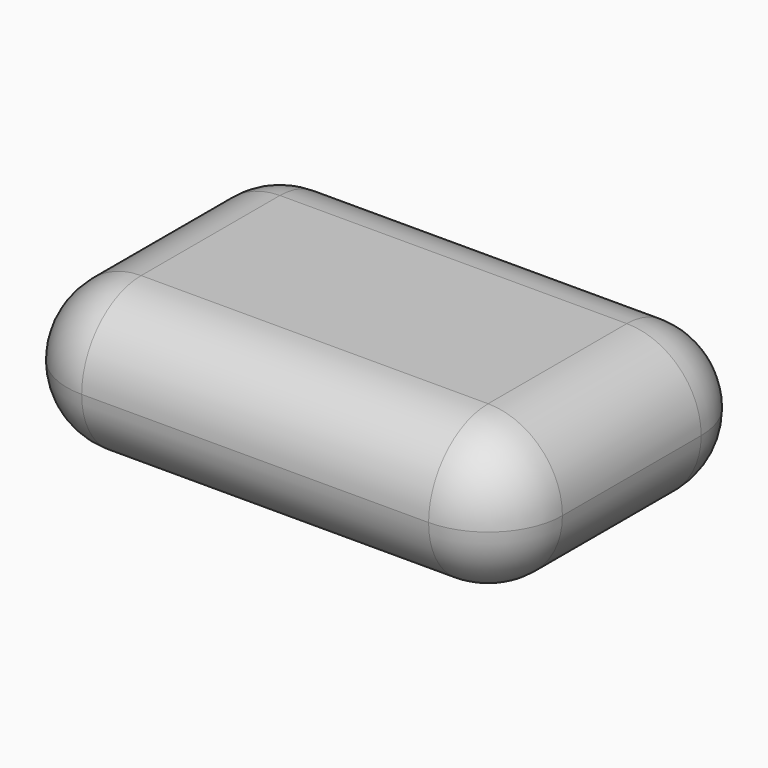
from build123d import *

# Parameters (mm, degrees)
F0_W     = 508
F0_H     = 330.2
F1_DEPTH = 152.4
F2_R     = 76.19999


# Not quite as in the source:
# - a fillet or chamfer is up to 0.001 mm smaller than in the source, because OpenCascade refuses the exact size


with BuildPart() as f1:
    # F0 (on Top) → F1 (new body)
    with BuildSketch(Plane.XY):
        Rectangle(F0_W, F0_H)
    extrude(amount=F1_DEPTH)

    # F2 (radius 76.2 in the source; OpenCascade refuses exactly that, so slightly less here)
    f2_edges = [f1.edges().sort_by_distance(p)[0] for p in [
        (254, 0, 152.4),
        (0, 165.1, 152.4),
        (-254, 0, 152.4),
        (0, -165.1, 152.4),
        (-254, -165.1, 76.2),
        (254, -165.1, 76.2),
        (0, -165.1, 0),
        (254, 165.1, 76.2),
        (254, 0, 0),
        (-254, 165.1, 76.2),
        (0, 165.1, 0),
        (-254, 0, 0),
    ]]
    fillet(f2_edges, radius=F2_R)


solid = f1.part
